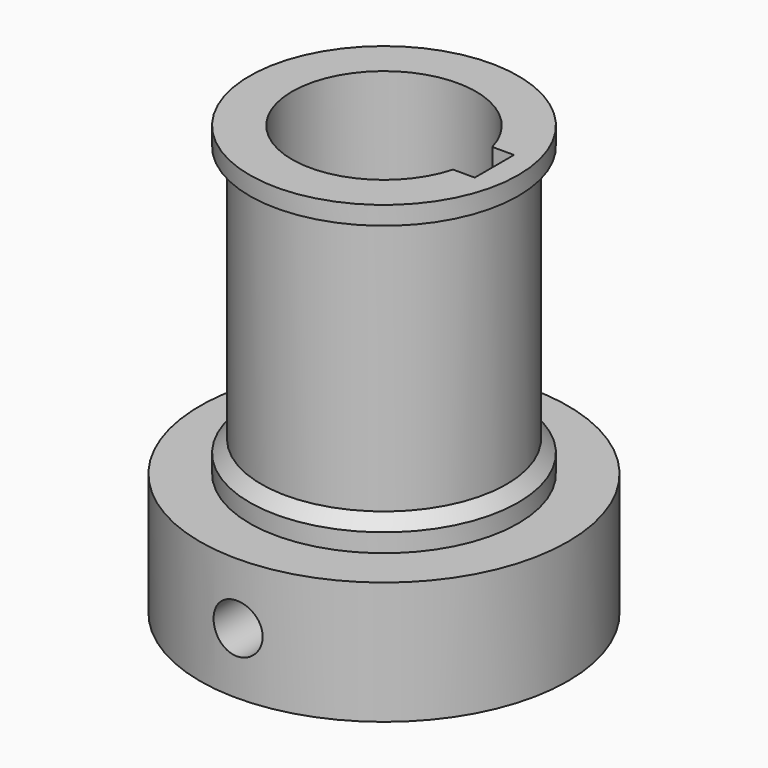
from build123d import *

# Parameters (mm, degrees)
F0_R      = 30
F1_DEPTH  = 20
F3_R      = 21.9
F4_DEPTH  = 3
F6_R      = 21.9
F7_DEPTH  = 2
F9_R      = 20
F10_DEPTH = 42
F11_SIZE2 = 1.99999
F11_SIZE  = 1.89999
F12_R     = 21.9
F13_DEPTH = 3
F15_DEPTH = 78
F16_R     = 4
F17_DEPTH = 45


# Not quite as in the source:
# - a fillet or chamfer is up to 0.001 mm smaller than in the source, because OpenCascade refuses the exact size


with BuildPart() as f1:
    # F0 (on Top) → F1 (new body)
    with BuildSketch(Plane.XY):
        Circle(F0_R)
    extrude(amount=F1_DEPTH)

    # F3 (on offset) → F4 (join)
    with BuildSketch(Plane.XY.offset(20)):
        Circle(F3_R)
    extrude(amount=F4_DEPTH)

    # F6 (on offset) → F7 (join)
    with BuildSketch(Plane.XY.offset(23)):
        Circle(F6_R)
    extrude(amount=F7_DEPTH)

    # F9 (on offset) → F10 (join)
    with BuildSketch(Plane.XY.offset(25)):
        Circle(F9_R)
    extrude(amount=F10_DEPTH)

    # F11 (size 1.9 and 2 in the source; OpenCascade refuses exactly that, so slightly less here)
    f11_edges = [f1.edges().sort_by_distance(p)[0] for p in [
        (-21.9, 0, 25),
    ]]
    f11_side = f1.faces().sort_by_distance((-21.280574, 0, 25))[0]
    chamfer(f11_edges, length=F11_SIZE, length2=F11_SIZE2, reference=f11_side)

    # F12 (on face) → F13 (join)
    with BuildSketch(Plane.XY.offset(67)):
        Circle(F12_R)
    extrude(amount=F13_DEPTH)

    # F14 (on face) → F15 (cut)
    with BuildSketch(Plane.XY.offset(70)):
        with BuildLine():
            Line((18, 4), (14.4568322948, 4))
            ThreePointArc((14.4568322948, 4), (-15, 0), (14.4568322948, -4))
            Line((14.4568322948, -4), (18, -4))
            Line((18, -4), (18, 0))
            Line((18, 0), (18, 4))
        make_face()
    extrude(amount=-F15_DEPTH, mode=Mode.SUBTRACT)

    # F16 (on Front) → F17 (cut)
    with BuildSketch(Plane.XZ):
        with Locations((0, 10)):
            Circle(F16_R)
    extrude(amount=F17_DEPTH, mode=Mode.SUBTRACT)


solid = f1.part
